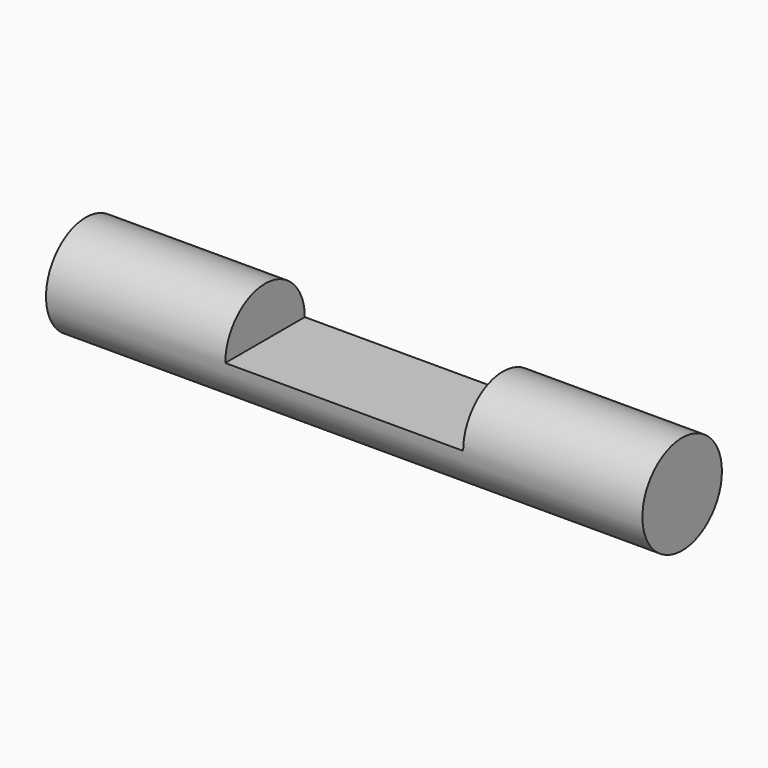
from build123d import *

# Parameters (mm, degrees)
F0_R     = 6.35
F1_DEPTH = 38.1
F2_W     = 30.3907971829
F2_H     = 7.0625422522
F3_DEPTH = 25.4


with BuildPart() as f1:
    # F0 (on Right) → F1 (new body, symmetric)
    with BuildSketch(Plane.YZ):
        Circle(F0_R)
    extrude(amount=F1_DEPTH, both=True)

    # F2 (on Front) → F3 (cut, symmetric)
    with BuildSketch(Plane.XZ):
        with Locations((0, 3.5312711261)):
            Rectangle(F2_W, F2_H)
    extrude(amount=F3_DEPTH, both=True, mode=Mode.SUBTRACT)


solid = f1.part
